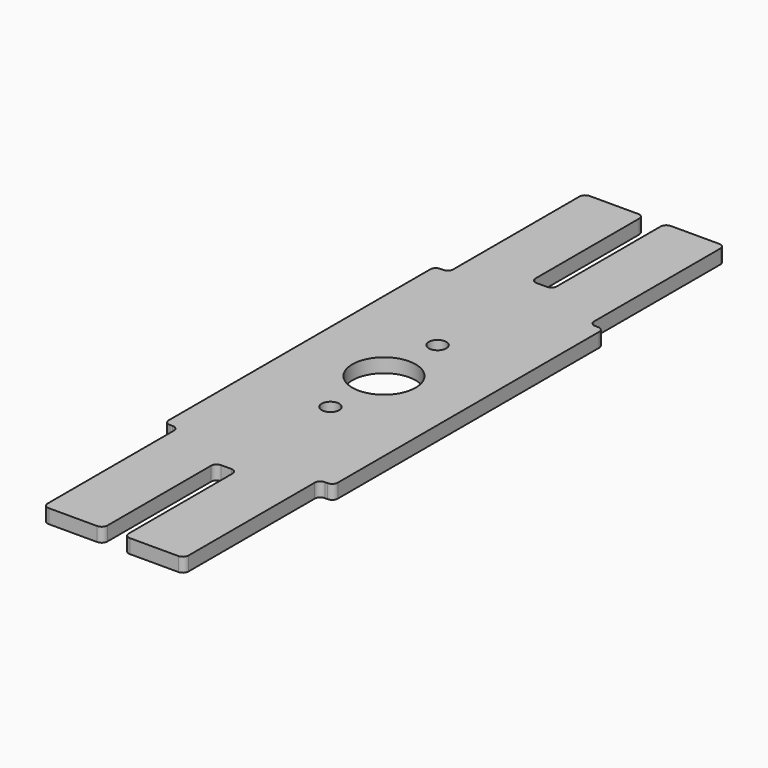
from build123d import *

# Parameters (mm, degrees)
F0_W     = 63.5
F0_H     = 304.8
F1_DEPTH = 6.35
F2_W     = 76.2
F2_H     = 152.4
F3_DEPTH = 6.35
F4_W     = 9.652
F4_H     = 63.5
F4_R     = 14.2875
F4_R_2   = 3.96875
F5_DEPTH = 6.351
F6_R     = 2.54


with BuildPart() as f1:
    # F0 (on Top) → F1 (new body)
    with BuildSketch(Plane.XY):
        Rectangle(F0_W, F0_H)
    extrude(amount=F1_DEPTH)

    # F2 (on Top) → F3 (join)
    with BuildSketch(Plane.XY):
        Rectangle(F2_W, F2_H)
    extrude(amount=F3_DEPTH)

    # F4 (on face) → F5 (cut, through all)
    with BuildSketch(Plane.XY.offset(6.35)):
        with Locations((0, 120.65)):
            Rectangle(F4_W, F4_H)
        with Locations((0, -120.65)):
            Rectangle(F4_W, F4_H)
        Circle(F4_R)
        with Locations((0, 30.1625)):
            Circle(F4_R_2)
        with Locations((0, -30.1625)):
            Circle(F4_R_2)
    extrude(amount=-F5_DEPTH, mode=Mode.SUBTRACT)

    # F6
    f6_edges = [f1.edges().sort_by_distance(p)[0] for p in [
        (-38.1, 76.2, 3.175),
        (-31.75, 76.2, 3.175),
        (-31.75, 152.4, 3.175),
        (-4.826, 152.4, 3.175),
        (4.826, 152.4, 3.175),
        (4.826, 88.9, 3.175),
        (-4.826, 88.9, 3.175),
        (31.75, 152.4, 3.175),
        (31.75, 76.2, 3.175),
        (38.1, 76.2, 3.175),
        (38.1, -76.2, 3.175),
        (31.75, -76.2, 3.175),
        (31.75, -152.4, 3.175),
        (4.826, -152.4, 3.175),
        (4.826, -88.9, 3.175),
        (-4.826, -88.9, 3.175),
        (-4.826, -152.4, 3.175),
        (-31.75, -152.4, 3.175),
        (-31.75, -76.2, 3.175),
        (-38.1, -76.2, 3.175),
    ]]
    fillet(f6_edges, radius=F6_R)


solid = f1.part
